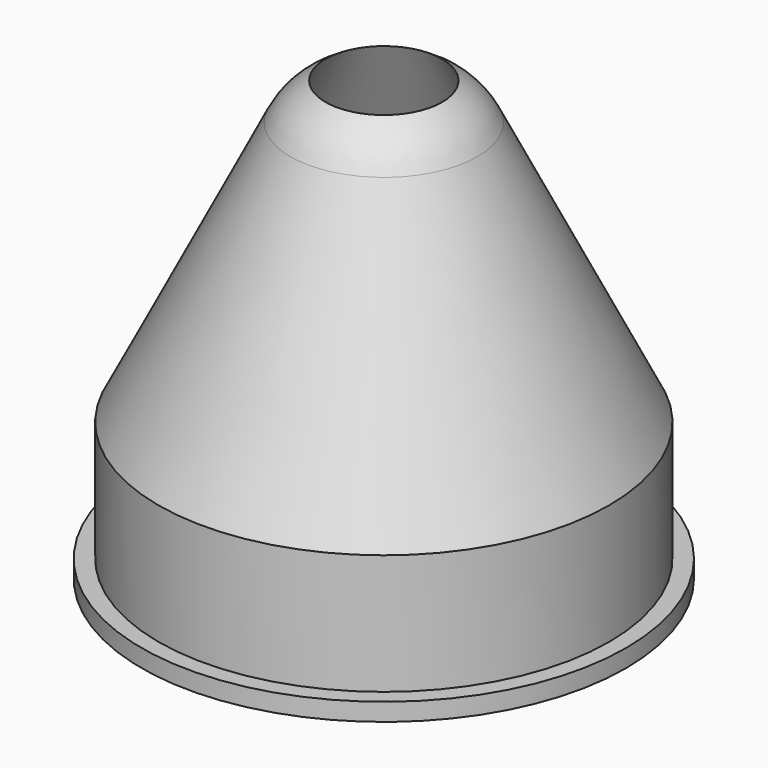
from build123d import *

# Parameters (mm, degrees)
F0_R      = 38.1
F0_R_2    = 34.29
F1_DEPTH  = 20.32
F4_R      = 38.1
F3_R      = 12.7
F6_T      = -2.54
F5_FACE_R = 34.29
F7_DEPTH  = 3.556
F7_TAPER  = 8
F9_R      = 40.932761629
F10_DEPTH = 3
F11_R     = 35.392761629
F12_DEPTH = 4.6


# Not quite as in the source:
# - a fillet or chamfer that OpenCascade refuses, or shapes differently, is made with other operations: its cross-section is extruded or revolved along the edge and cut away or added


with BuildPart() as f1:
    # F0 (on Top) → F1 (new body)
    with BuildSketch(Plane.XY):
        Circle(F0_R)
        Circle(F0_R_2, mode=Mode.SUBTRACT)
    extrude(amount=F1_DEPTH)

    # F4 (on face) → F5 section 0
    with BuildSketch(Plane.XY.offset(20.32)):
        Circle(F4_R)
    # F3 (on offset) → F5 section 1
    with BuildSketch(Plane.XY.offset(71.12)):
        Circle(F3_R)
    loft()

    # F6
    f6_openings = [f1.faces().sort_by_distance(p)[0] for p in [
        (0, 0, 71.12),
    ]]
    offset(amount=F6_T, openings=f6_openings, kind=Kind.INTERSECTION)

    # F5_face (on face) → F7 (cut)
    with BuildSketch(Plane(origin=(0, 0, 20.32), x_dir=(1, 0, 0), z_dir=(0, 0, -1))):
        Circle(F5_FACE_R)
    extrude(amount=-F7_DEPTH, taper=F7_TAPER, mode=Mode.SUBTRACT)

    # F8: fillet of radius 14.4671225158 on 1 edges, made by hand

    # F8_s1 → F8_t2 (revolve, cut)
    with BuildSketch(Plane.XZ):
        with BuildLine():
            ThreePointArc((15.7937700832, 64.9324598335), (13.2958276301, 68.4758321875), (9.8601936686, 71.12))
            Line((9.8601936686, 71.12), (12.7, 71.12))
            Line((12.7, 71.12), (15.7937700832, 64.9324598335))
        make_face()
    revolve(axis=Axis((0, 0, 71.12), (0, 0, 1)), mode=Mode.SUBTRACT)

    # F9 (on Top) → F10 (join)
    with BuildSketch(Plane.XY):
        Circle(F9_R)
    extrude(amount=-F10_DEPTH)

    # F11 (on face) → F12 (cut)
    with BuildSketch(Plane(origin=(0, 0, -3), x_dir=(1, 0, 0), z_dir=(0, 0, -1))):
        Circle(F11_R)
    extrude(amount=-F12_DEPTH, mode=Mode.SUBTRACT)


solid = f1.part
